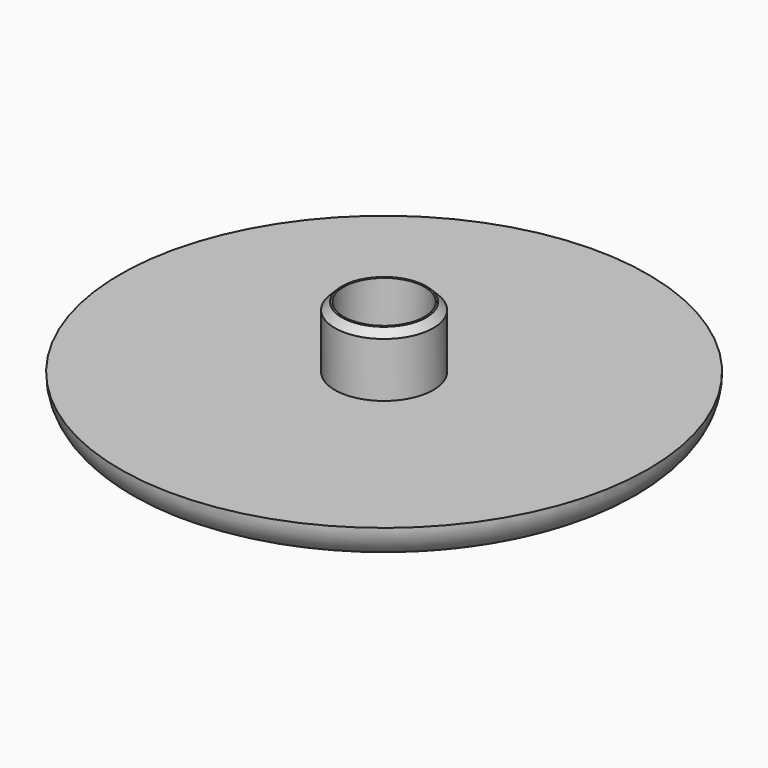
from build123d import *

# Parameters (mm, degrees)
F0_R      = 2.8
F1_DEPTH  = 3.5
F2_T      = -0.5
F0_R_2    = 15
F1_FACE_R = 2.8
F3_DEPTH  = 2
F4_R      = 1.99999
F5_SIZE   = 0.4


# Not quite as in the source:
# - a fillet or chamfer is up to 0.001 mm smaller than in the source, because OpenCascade refuses the exact size


with BuildPart() as f1:
    # F0 (on Top) → F1 (new body)
    with BuildSketch(Plane.XY):
        Circle(F0_R)
    extrude(amount=F1_DEPTH)

    # F2
    f2_openings = [f1.faces().sort_by_distance(p)[0] for p in [
        (0, 0, 3.5),
    ]]
    offset(amount=F2_T, openings=f2_openings)

    # F0 (on Top) + F1_face (on face) → F3 (join)
    with BuildSketch(Plane.XY):
        Circle(F0_R_2)
        Circle(F0_R, mode=Mode.SUBTRACT)
    with BuildSketch(Plane(origin=(0, 0, 0), x_dir=(1, 0, 0), z_dir=(0, 0, -1))):
        Circle(F1_FACE_R)
    extrude(amount=-F3_DEPTH, dir=(0, 0, 1))

    # F4 (radius 2 in the source; OpenCascade refuses exactly that, so slightly less here)
    f4_edges = [f1.edges().sort_by_distance(p)[0] for p in [
        (-15, 0, -2),
    ]]
    fillet(f4_edges, radius=F4_R)

    # F5
    f5_edges = [f1.edges().sort_by_distance(p)[0] for p in [
        (-2.8, 0, 3.5),
    ]]
    chamfer(f5_edges, length=F5_SIZE)


solid = f1.part
